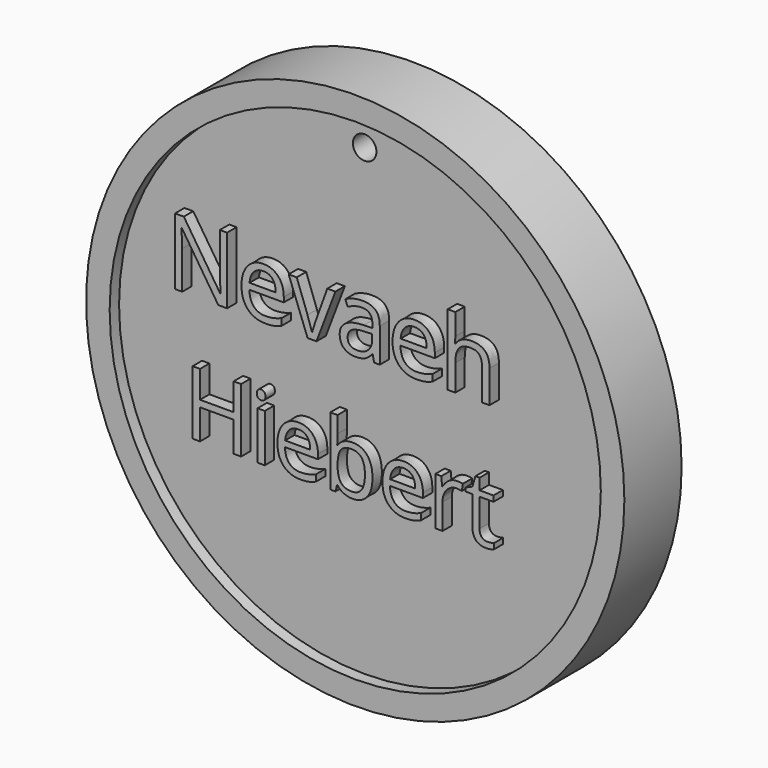
from build123d import *

# Parameters (mm, degrees)
F0_R         = 57.15
F1_DEPTH     = 6.35
F3_R         = 57.15
F3_R_2       = 52.1499998868
F4_DEPTH     = 2.5
F8_D         = 5
F5_TEXT_SIZE = 19.8230088496
F9_DEPTH     = 2.5
F6_TEXT_SIZE = 18.9914465106
F10_DEPTH    = 2.5


# Not quite as in the source:
# - Text() gives the source's letters only with a copy of the font that has no kerning and outlines rounded to 1/6400 em; it was checked with that copy


with BuildPart() as f1:
    # F0 (on Front) → F1 (new body, symmetric)
    with BuildSketch(Plane.XZ):
        Circle(F0_R)
    extrude(amount=F1_DEPTH, both=True)

    # F3 (on face) → F4 (join)
    with BuildSketch(Plane.XZ.offset(6.35)):
        Circle(F3_R)
        Circle(F3_R_2, mode=Mode.SUBTRACT)
    extrude(amount=F4_DEPTH)

    # F8 (through all)
    with Locations(Plane.XZ.offset(6.35)):
        with Locations((0, 46.2714023888)):
            Hole(F8_D / 2)

    # F5 (on face) → F9 (join)
    with BuildSketch(Plane.XZ.offset(6.35)):
        with Locations((-40.2063503861, 8.3803614144)):
            Text('Nevaeh', F5_TEXT_SIZE, font='Open Sans', text_align=(TextAlign.LEFT, TextAlign.BOTTOM))
    extrude(amount=F9_DEPTH)

    # F6 (on face) → F10 (join)
    with BuildSketch(Plane.XZ.offset(6.35)):
        with Locations((-36.3974012434, -18.368627876)):
            Text('Hiebert', F6_TEXT_SIZE, font='Open Sans', text_align=(TextAlign.LEFT, TextAlign.BOTTOM))
    extrude(amount=F10_DEPTH)


solid = f1.part
